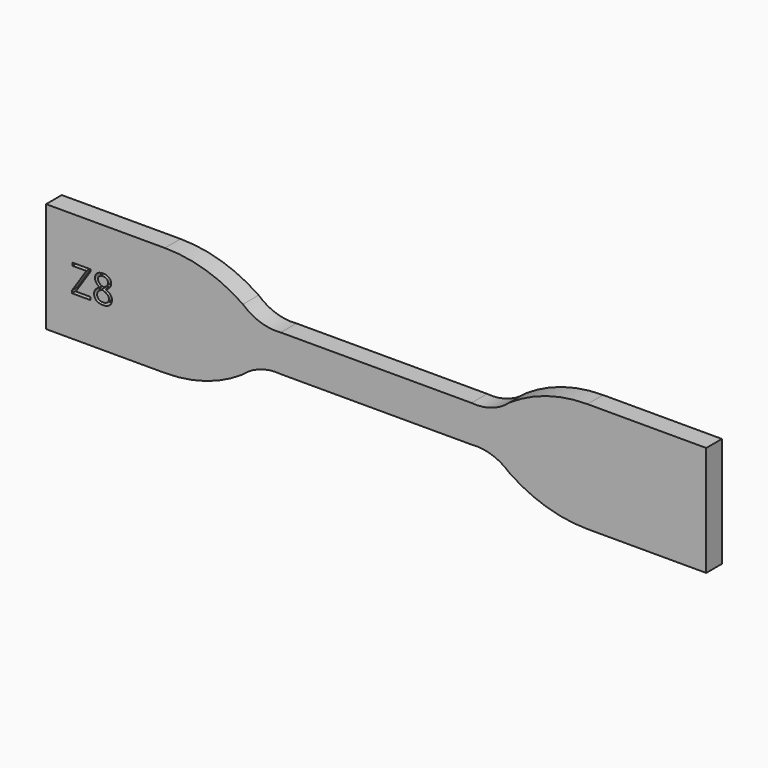
from build123d import *

# Parameters (mm, degrees)
F1_DEPTH     = 3.3999932
F2_TEXT_SIZE = 6.5938345051
F3_DEPTH     = 1.27


# Not quite as in the source:
# - Text() gives the source's letters only with a copy of the font that has no kerning and outlines rounded to 1/6400 em; it was checked with that copy


with BuildPart() as f1:
    # F0 (on Front) → F1 (new body)
    with BuildSketch(Plane.XZ):
        with BuildLine():
            Line((-57.15, 9.525), (-57.15, 0))
            Line((-57.15, 0), (-57.15, -9.525))
            Line((-57.15, -9.525), (-36.5849584341, -9.525))
            ThreePointArc((-36.5849584341, -9.525), (-29.510865085, -8.4575375348), (-23.0667367578, -5.3502102382))
            ThreePointArc((-23.0667367578, -5.3502102382), (-20.0158934059, -3.5767763741), (-16.51, -3.175))
            Line((-16.51, -3.175), (0, -3.175))
            Line((0, -3.175), (16.51, -3.175))
            ThreePointArc((16.51, -3.175), (20.0158934059, -3.5767763741), (23.0667367578, -5.3502102382))
            ThreePointArc((23.0667367578, -5.3502102382), (29.510865085, -8.4575375348), (36.5849584341, -9.525))
            Line((36.5849584341, -9.525), (57.15, -9.525))
            Line((57.15, -9.525), (57.15, 0))
            Line((57.15, 0), (57.15, 9.525))
            Line((57.15, 9.525), (36.5849584341, 9.525))
            ThreePointArc((36.5849584341, 9.525), (29.510865085, 8.4575375348), (23.0667367578, 5.3502102382))
            ThreePointArc((23.0667367578, 5.3502102382), (20.0158934059, 3.5767763741), (16.51, 3.175))
            Line((16.51, 3.175), (0, 3.175))
            Line((0, 3.175), (-16.51, 3.175))
            ThreePointArc((-16.51, 3.175), (-20.0158934059, 3.5767763741), (-23.0667367578, 5.3502102382))
            ThreePointArc((-23.0667367578, 5.3502102382), (-29.510865085, 8.4575375348), (-36.5849584341, 9.525))
            Line((-36.5849584341, 9.525), (-57.15, 9.525))
        make_face()
    extrude(amount=F1_DEPTH)

    # F2 (on face) → F3 (cut)
    with BuildSketch(Plane.XZ.offset(3.3999932)):
        with Locations((-52.9304846442, -2.6073189134)):
            Text('Z8', F2_TEXT_SIZE, font='Open Sans', text_align=(TextAlign.LEFT, TextAlign.BOTTOM))
    extrude(amount=-F3_DEPTH, mode=Mode.SUBTRACT)


solid = f1.part
